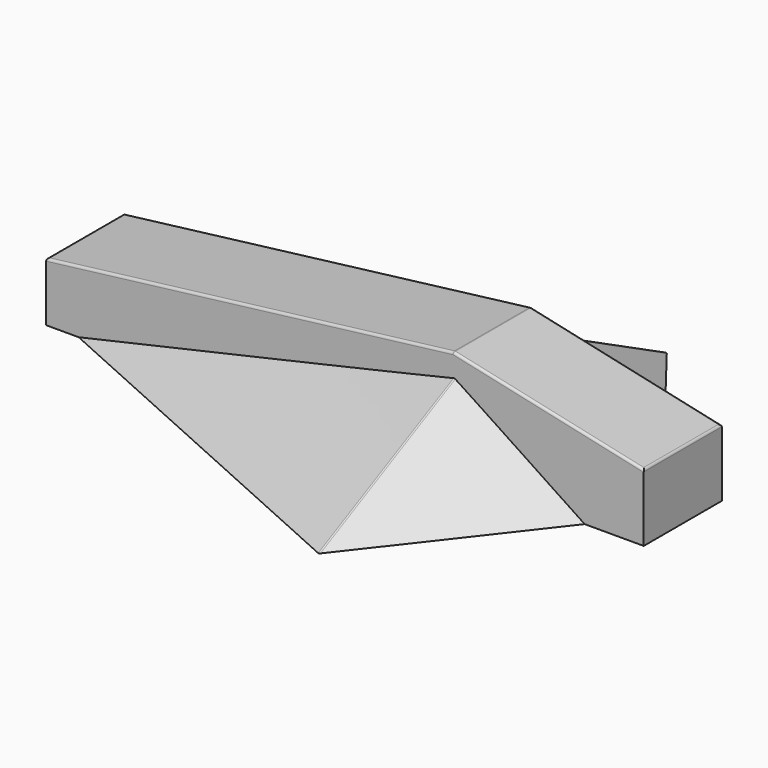
from build123d import *

# Parameters (mm, degrees)
F5_DEPTH = 600
F7_DEPTH = 1469.6233856019
F8_R     = 13


with BuildPart() as f3:
    # F0 (on Top) → F3 section 0
    with BuildSketch(Plane.XY):
        Polygon((1800, 0), (868.0580854416, 1200), (-1800, 0), (868.0580854416, -1200), align=None)
    # F2 (on offset) → F3 section 1
    with BuildSketch(Plane.XY.offset(600)):
        Polygon((899.0031123161, 0), (874.0031123161, 25), (849.0031123161, 0), (874.0031123161, -25), align=None)
    loft()

    # F4 (on face) → F5 (join)
    with BuildSketch(Plane.XY):
        Polygon((-1200.5265119548, -269.6223855019), (1590.6063315397, -269.6223855019), (1800, 0), (1590.6063315397, 269.6223855019), (-1200.5265119548, 269.6223855019), (-1800, 0), align=None)
        Polygon((-1916.4335727692, -269.6223855019), (-1200.5265119548, -269.6223855019), (-1800, 0), (-1200.5265119548, 269.6223855019), (-1916.4335727692, 269.6223855019), align=None)
        Polygon((1590.6063315397, -269.6223855019), (1916.4335727692, -269.6223855019), (1916.4335727692, 269.6223855019), (1590.6063315397, 269.6223855019), (1800, 0), align=None)
    extrude(amount=F5_DEPTH)

    # F6 (on face) → F7 (cut, through all)
    with BuildSketch(Plane.XZ.offset(269.6223855019)):
        Polygon((-1380.3998167432, 323.7263331278), (865.4105067253, 600), (-1916.4335727692, 600), (-1916.4335727692, 0), (-1380.3998167432, 0), align=None)
        Polygon((1916.4335727692, 600), (865.4105067253, 600), (1916.4335727692, 370.3585863113), align=None)
    extrude(amount=-F7_DEPTH, mode=Mode.SUBTRACT)

    # F8
    f8_edges = [f3.edges().sort_by_distance(p)[0] for p in [
        (1390.92204, -269.622386, 485.179293),
        (1916.433573, 0, 370.358586),
        (-257.494655, -269.622386, 461.863167),
        (865.410507, 0, 600),
        (-257.494655, 269.622386, 461.863167),
        (-1380.399817, 0, 323.726333),
        (1390.92204, 269.622386, 485.179293),
        (870.411753, -734.811193, 237.543221),
        (870.411753, 734.811193, 237.543221),
    ]]
    fillet(f8_edges, radius=F8_R)


solid = f3.part
